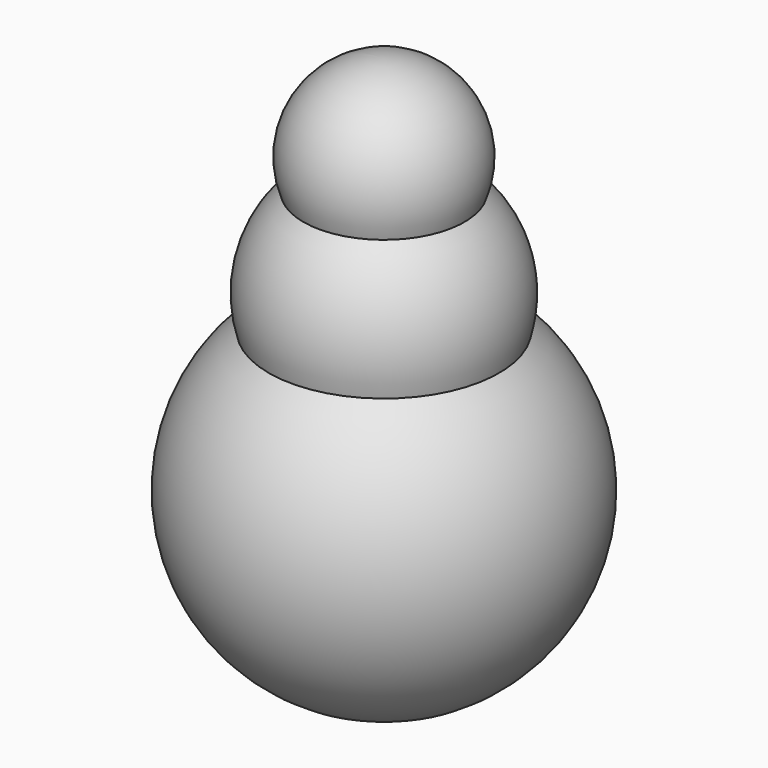
from build123d import *


with BuildPart() as f1:
    # F0 (on Front) → F1 (revolve)
    with BuildSketch(Plane.XZ):
        with BuildLine():
            Line((0, 25.9262488724), (0, 44.637852612))
            ThreePointArc((0, 44.637852612), (-15.4348737394, 36.5039984988), (-17.4508002843, 19.1739393457))
            ThreePointArc((-17.4508002843, 19.1739393457), (-9.3558018698, 24.179316615), (0, 25.9262488724))
        make_face()
        with BuildLine():
            ThreePointArc((0, 7.2146451328), (-10.5777496264, 10.491375133), (-17.4508002843, 19.1739393457))
            ThreePointArc((-17.4508002843, 19.1739393457), (-24.945118357, 7.0648036597), (-24.9134138156, -7.1758060625))
            ThreePointArc((-24.9134138156, -7.1758060625), (-13.2302178856, -0.5567017681), (0, 1.7391517758))
            Line((0, 1.7391517758), (0, 7.2146451328))
        make_face()
        with BuildLine():
            ThreePointArc((0, -25.9262488724), (-15.590520305, -20.7148752643), (-24.9134138156, -7.1758060625))
            ThreePointArc((-24.9134138156, -7.1758060625), (-36.9726810866, -50.7596007403), (0, -76.7979174852))
            Line((0, -76.7979174852), (0, -25.9262488724))
        make_face()
        with BuildLine():
            ThreePointArc((0, 1.7391517758), (-13.2302178856, -0.5567017681), (-24.9134138156, -7.1758060625))
            ThreePointArc((-24.9134138156, -7.1758060625), (-15.590520305, -20.7148752643), (0, -25.9262488724))
            Line((0, -25.9262488724), (0, 1.7391517758))
        make_face()
        with BuildLine():
            Line((0, 7.2146451328), (0, 25.9262488724))
            ThreePointArc((0, 25.9262488724), (-9.3558018698, 24.179316615), (-17.4508002843, 19.1739393457))
            ThreePointArc((-17.4508002843, 19.1739393457), (-10.5777496264, 10.491375133), (0, 7.2146451328))
        make_face()
    revolve(axis=Axis((0, 0, -5.5481381714), (0, 0, -1)))


solid = f1.part
